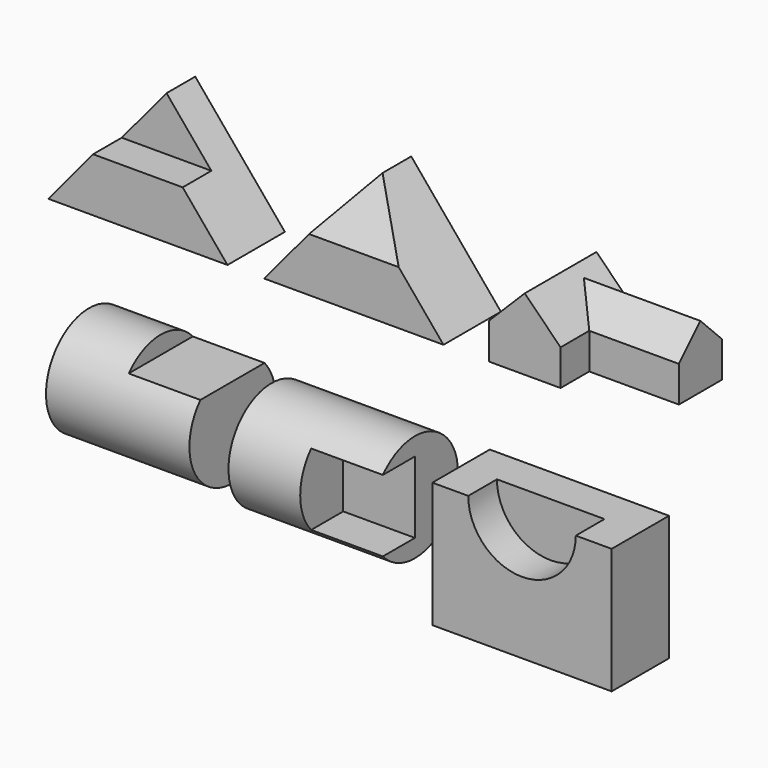
from build123d import *

# Parameters (mm, degrees)
F1_DEPTH  = 101.6
F3_DEPTH  = 50.8
F5_DEPTH  = 101.6
F9_DEPTH  = 63.5
F11_DEPTH = 127
F15_R     = 76.2
F16_DEPTH = 203.2
F18_DEPTH = 101.6
F20_R     = 76.2
F21_DEPTH = 203.2
F23_DEPTH = 101.6
F24_W     = 254
F24_H     = 177.8
F25_DEPTH = 101.6
F27_DEPTH = 50.8


# Not quite as in the source:
# - a feature names something its author has since deleted; it is built from what else it names


with BuildPart() as f1:
    # F0 (on Front) → F1 (new body)
    with BuildSketch(Plane.XZ):
        Polygon((63.5, 76.2), (190.5, 76.2), (127, 152.4), align=None)
        Polygon((0, 0), (254, 0), (190.5, 76.2), (63.5, 76.2), align=None)
    extrude(amount=-F1_DEPTH)

    # F2 (on face) → F3 (cut)
    with BuildSketch(Plane.XZ):
        Polygon((127, 76.2), (127, 152.4), (63.5, 76.2), align=None)
        Polygon((190.5, 76.2), (127, 152.4), (127, 76.2), align=None)
    extrude(amount=-F3_DEPTH, mode=Mode.SUBTRACT)


with BuildPart() as f5:
    # F4 (on face) → F5 (new body)
    with BuildSketch(Plane.XZ):
        Polygon((306.055911541, 0), (560.055911541, 0), (433.055911541, 152.4), align=None)
    extrude(amount=-F5_DEPTH)

    # F8 (on 3pt) → F9 (cut, symmetric)
    with BuildSketch(Plane.YZ.offset(433.055911541)):
        Polygon((50.8, 152.4), (0, 152.4), (0, 76.2), align=None)
    extrude(amount=F9_DEPTH, both=True, mode=Mode.SUBTRACT)


with BuildPart() as f11:
    # F10 (on face) → F11 (new body)
    with BuildSketch(Plane.XZ):
        Polygon((675.1348665619, 101.6), (624.3348665619, 50.8), (624.3348665619, 0), (725.9348665619, 0), (725.9348665619, 50.8), align=None)
    extrude(amount=-F11_DEPTH)

    # F13 (on offset) → F14 (join, up to the next surface of F11)
    with BuildSketch(Plane.YZ.offset(852.9348665619)):
        Polygon((50.8, 50.8), (50.8, 0), (127, 0), (127, 50.8), (88.9, 88.9), align=None)
    extrude(until=Until.NEXT, dir=(-1, 0, 0))


with BuildPart() as f16:
    # F15 (on Right) → F16 (new body)
    with BuildSketch(Plane.YZ):
        with Locations((72.2502991557, -241.928935051)):
            Circle(F15_R)
    extrude(amount=F16_DEPTH)

    # F17 (on face) → F18 (cut)
    with BuildSketch(Plane.YZ.offset(203.2)):
        with BuildLine():
            ThreePointArc((129.0464257842, -191.128935051), (72.2502991557, -165.728935051), (15.4541725272, -191.128935051))
            Line((15.4541725272, -191.128935051), (129.0464257842, -191.128935051))
        make_face()
    extrude(amount=-F18_DEPTH, mode=Mode.SUBTRACT)


with BuildPart() as f21:
    # F20 (on offset) → F21 (new body)
    with BuildSketch(Plane.YZ.offset(266.7)):
        with Locations((62.1099583805, -244.6303920269)):
            Circle(F20_R)
    extrude(amount=F21_DEPTH)

    # F22 (on face) → F23 (cut)
    with BuildSketch(Plane.YZ.offset(469.9)):
        with BuildLine():
            Line((5.313831752, -295.4303920269), (62.1099583805, -295.4303920269))
            Line((62.1099583805, -295.4303920269), (62.1099583805, -244.6303920269))
            Line((62.1099583805, -244.6303920269), (62.1099583805, -193.8303920269))
            Line((62.1099583805, -193.8303920269), (5.313831752, -193.8303920269))
            ThreePointArc((5.313831752, -193.8303920269), (-14.0900416195, -244.6303920269), (5.313831752, -295.4303920269))
        make_face()
    extrude(amount=-F23_DEPTH, mode=Mode.SUBTRACT)


with BuildPart() as f25:
    # F24 (on face) → F25 (new body)
    with BuildSketch(Plane.XZ.offset(-62.1099583805)):
        with Locations((702.8850913048, -239.6382312099)):
            Rectangle(F24_W, F24_H)
    extrude(amount=F25_DEPTH)

    # F26 (on face) → F27 (cut)
    with BuildSketch(Plane.XZ.offset(39.4900416195)):
        with BuildLine():
            Line((779.0850913048, -150.7382312099), (626.6850913048, -150.7382312099))
            ThreePointArc((626.6850913048, -150.7382312099), (702.8850913048, -226.9382312099), (779.0850913048, -150.7382312099))
        make_face()
    extrude(amount=-F27_DEPTH, mode=Mode.SUBTRACT)


solid = Compound([f1.part, f5.part, f11.part, f16.part, f21.part, f25.part])
